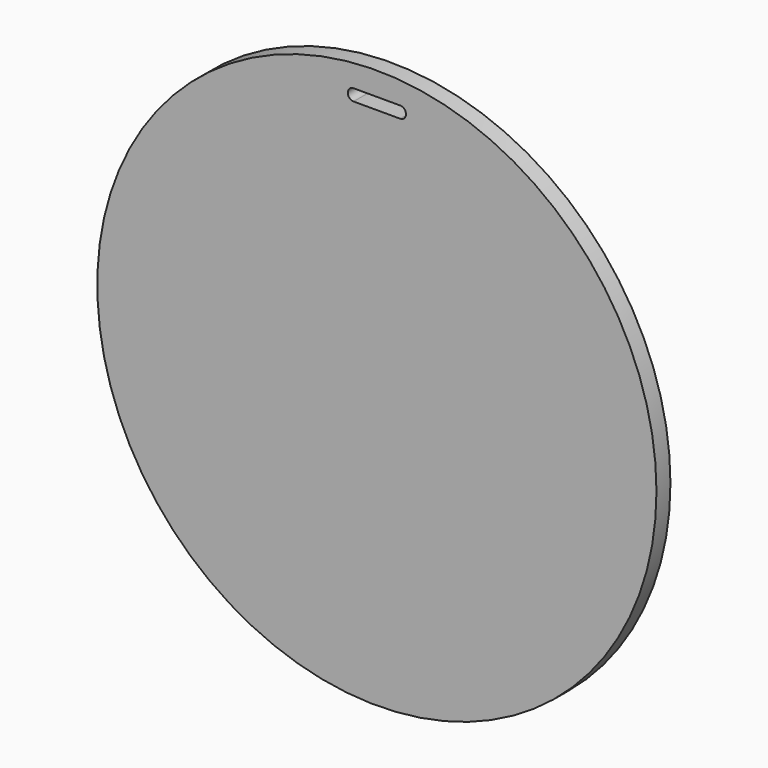
from build123d import *

# Parameters (mm, degrees)
F1_DEPTH = 9.525


# Not quite as in the source:
# - a length typed as a fraction of an inch, garbled in the dataset ("3 / 203.2 mm" for 3/8 in), is restored


with BuildPart() as f1:
    # F0 (on Front) → F1 (new body)
    with BuildSketch(Plane.XZ):
        with BuildLine():
            ThreePointArc((0, 152.4), (-107.7630734528, -107.7630734528), (152.4, 0))
            ThreePointArc((152.4, 0), (107.7630734528, 107.7630734528), (0, 152.4))
        make_face()
        with BuildLine():
            Line((-12.7, 139.7), (0, 139.7))
            Line((0, 139.7), (12.7, 139.7))
            ThreePointArc((12.7, 139.7), (14.9450640303, 138.7700640303), (15.875, 136.525))
            ThreePointArc((15.875, 136.525), (14.9450640303, 134.2799359697), (12.7, 133.35))
            Line((12.7, 133.35), (0, 133.35))
            Line((0, 133.35), (-12.7, 133.35))
            ThreePointArc((-12.7, 133.35), (-15.875, 136.525), (-12.7, 139.7))
        make_face(mode=Mode.SUBTRACT)
    extrude(amount=F1_DEPTH)


solid = f1.part
